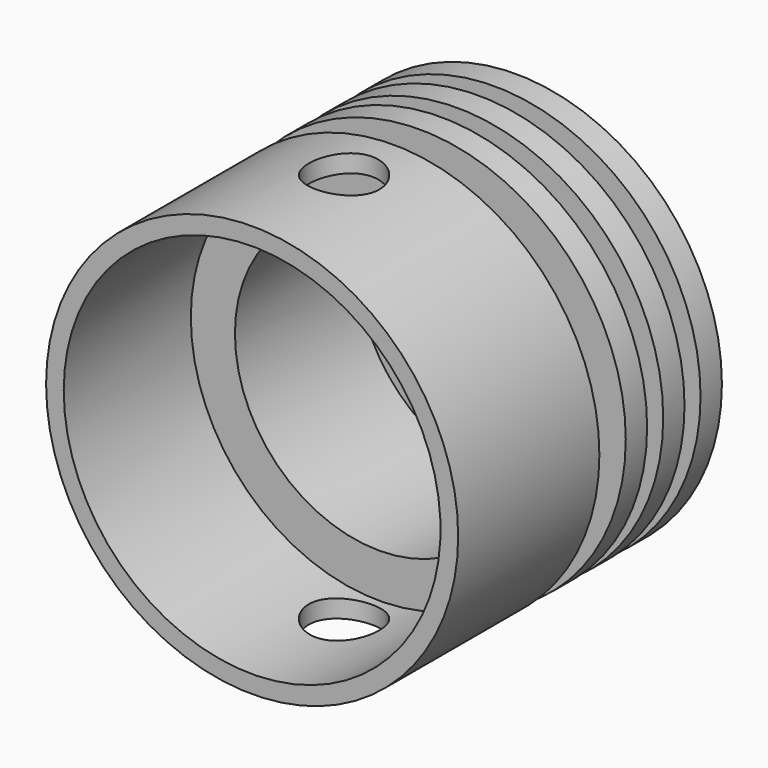
from build123d import *

# Parameters (mm, degrees)
F2_T     = 3.175
F3_R     = 6.35
F4_DEPTH = 64.008
F5_DEPTH = 104.14


# Not quite as in the source:
# - a shell that OpenCascade refuses in one call is made with other operations: the cavity is built on its own and cut out


with BuildPart() as f1:
    # F0 (on Top) → F1 (revolve)
    with BuildSketch(Plane.XY):
        Polygon((-37.0614958425, 0), (0, 0), (0, 59.2983933481), (-37.0614958425, 59.2983933481), (-37.0614958425, 54.4952234869), (-29.1296224819, 54.4952234869), (-29.1296224819, 50.8915618087), (-37.0614958425, 50.8915618087), (-37.0614958425, 46.1002111902), (-29.1296224819, 46.1002111902), (-29.1296224819, 42.483009196), (-37.0614958425, 42.483009196), (-37.0614958425, 37.6798393348), (-29.1296224819, 37.6798393348), (-29.1296224819, 31.75), (-37.0614958425, 31.75), align=None)
    revolve(axis=Axis((0, 29.649196674, 0), (0, 1, 0)))

    # F2: shell of thickness 3.175, made by hand


with BuildPart() as f2_core1:
    # F2_t2: copy of F1
    add(f1.part)

    # the walls: a layer under each face that stays
    f2_faces = [f2_core1.faces().sort_by_distance(p)[0] for p in [
        (29.1296224819, 34.7149196674, 0),
        (-24.707663895, 31.75, -24.707663895),
        (37.0614958425, 15.875, 0),
        (0, 59.2983933481, 0),
        (37.0614958425, 56.8968084175, 0),
        (24.707663895, 54.4952234869, -24.707663895),
        (29.1296224819, 52.6933926478, 0),
        (-24.707663895, 50.8915618087, -24.707663895),
        (37.0614958425, 48.4958864995, 0),
        (24.707663895, 46.1002111902, -24.707663895),
        (29.1296224819, 44.2916101931, 0),
        (-24.707663895, 42.483009196, -24.707663895),
        (37.0614958425, 40.0814242654, 0),
        (24.707663895, 37.6798393348, -24.707663895),
    ]]
    thicken(f2_faces, amount=-F2_T, mode=Mode.SUBTRACT)

    # F2_s3 → F2_t4 (revolve, cut)
    with BuildSketch(Plane.XY):
        Polygon((-29.1613724819, 37.6480893348), (-25.9546224819, 37.6798393348), (-25.9546224819, 40.8548393348), (-29.1296224819, 40.8548393348), align=None)
    revolve(axis=Axis((0, 37.6798393348, 0), (0, 1, 0)), mode=Mode.SUBTRACT)

    # F2_s5 → F2_t6 (revolve, cut)
    with BuildSketch(Plane.XY):
        Polygon((-29.1613724819, 31.78175), (-25.9546224819, 31.75), (-25.9546224819, 28.575), (-29.1296224819, 28.575), align=None)
    revolve(axis=Axis((0, 31.75, 0), (0, 1, 0)), mode=Mode.SUBTRACT)

    # F2_s7 → F2_t8 (revolve, cut)
    with BuildSketch(Plane.XY):
        Polygon((-29.1613724819, 54.4634734869), (-29.1296224819, 57.6702234869), (-25.9546224819, 57.6702234869), (-25.9546224819, 54.4952234869), align=None)
    revolve(axis=Axis((0, 54.4952234869, 0), (0, 1, 0)), mode=Mode.SUBTRACT)

    # F2_s9 → F2_t10 (revolve, cut)
    with BuildSketch(Plane.XY):
        Polygon((-29.1613724819, 50.9233118087), (-25.9546224819, 50.8915618087), (-25.9546224819, 47.7165618087), (-29.1296224819, 47.7165618087), align=None)
    revolve(axis=Axis((0, 50.8915618087, 0), (0, 1, 0)), mode=Mode.SUBTRACT)

    # F2_s11 → F2_t12 (revolve, cut)
    with BuildSketch(Plane.XY):
        Polygon((-29.1613724819, 46.0684611902), (-29.1296224819, 49.2752111902), (-25.9546224819, 49.2752111902), (-25.9546224819, 46.1002111902), align=None)
    revolve(axis=Axis((0, 46.1002111902, 0), (0, 1, 0)), mode=Mode.SUBTRACT)

    # F2_s13 → F2_t14 (revolve, cut)
    with BuildSketch(Plane.XY):
        Polygon((-29.1613724819, 42.514759196), (-25.9546224819, 42.483009196), (-25.9546224819, 39.308009196), (-29.1296224819, 39.308009196), align=None)
    revolve(axis=Axis((0, 42.483009196, 0), (0, 1, 0)), mode=Mode.SUBTRACT)


with BuildPart() as f1_1:
    add(f1.part)

    # what is left inside the walls is the cavity
    f2_cavity = [f2_core1.part.solids().sort_by_distance(p)[0] for p in [
        (33.854746, 19.05, 0),
    ]]
    add(f2_cavity, mode=Mode.SUBTRACT)

    # F3 (on Top) → F4 (cut)
    with BuildSketch(Plane.XY):
        with Locations((0, 20.6699799746)):
            Circle(F3_R)
    extrude(amount=-F4_DEPTH, mode=Mode.SUBTRACT)

    # F3 (on Top) → F5 (cut)
    with BuildSketch(Plane.XY):
        with Locations((0, 20.6699799746)):
            Circle(F3_R)
    extrude(amount=F5_DEPTH, mode=Mode.SUBTRACT)


solid = f1_1.part
